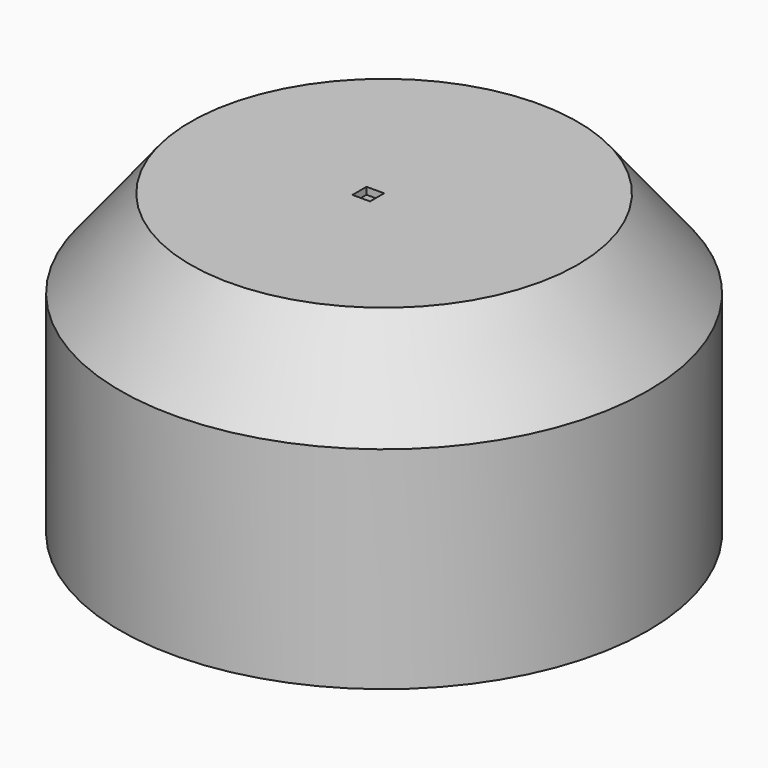
from build123d import *

# Parameters (mm, degrees)
F0_R     = 75
F1_DEPTH = 85
F2_SIZE2 = 25
F2_SIZE  = 20
F3_T     = -2
F4_W     = 5
F4_H     = 5
F5_DEPTH = 85.001


# Not quite as in the source:
# - the program builds the solid bodies; features that only make, move or delete a surface that nothing else refers to are left out


with BuildPart() as f1:
    # F0 (on Top) → F1 (new body)
    with BuildSketch(Plane.XY):
        Circle(F0_R)
    extrude(amount=F1_DEPTH)

    # F2
    f2_edges = [f1.edges().sort_by_distance(p)[0] for p in [
        (-75, 0, 85),
    ]]
    f2_side = f1.faces().sort_by_distance((0, 0, 85))[0]
    chamfer(f2_edges, length=F2_SIZE, length2=F2_SIZE2, reference=f2_side)

    # F3
    f3_openings = [f1.faces().sort_by_distance(p)[0] for p in [
        (0, 0, 0),
    ]]
    offset(amount=F3_T, openings=f3_openings)

    # F4 (on face) → F5 (cut, through all)
    with BuildSketch(Plane.XY.offset(85)):
        with Locations((-2.5, -2.5)):
            Rectangle(F4_W, F4_H)
    extrude(amount=-F5_DEPTH, mode=Mode.SUBTRACT)


solid = f1.part
